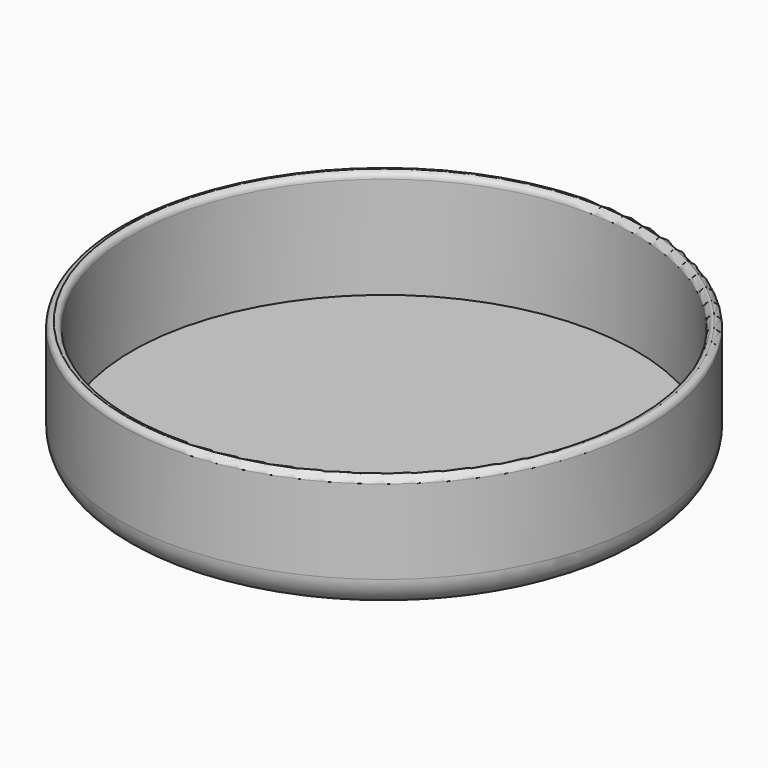
from build123d import *

# Parameters (mm, degrees)
F0_R     = 44
F1_DEPTH = 20
F2_T     = -2
F3_R     = 1
F4_R     = 0.99999
F5_R     = 5


# Not quite as in the source:
# - a fillet or chamfer is up to 0.001 mm smaller than in the source, because OpenCascade refuses the exact size


with BuildPart() as f1:
    # F0 (on Top) → F1 (new body)
    with BuildSketch(Plane.XY):
        Circle(F0_R)
    extrude(amount=F1_DEPTH)

    # F2
    f2_openings = [f1.faces().sort_by_distance(p)[0] for p in [
        (0, 0, 20),
    ]]
    offset(amount=F2_T, openings=f2_openings)

    # F3
    f3_edges = [f1.edges().sort_by_distance(p)[0] for p in [
        (-42, 0, 20),
    ]]
    fillet(f3_edges, radius=F3_R)

    # F4 (radius 1 in the source; OpenCascade refuses exactly that, so slightly less here)
    f4_edges = [f1.edges().sort_by_distance(p)[0] for p in [
        (-44, 0, 20),
    ]]
    fillet(f4_edges, radius=F4_R)

    # F5
    f5_edges = [f1.edges().sort_by_distance(p)[0] for p in [
        (-44, 0, 0),
    ]]
    fillet(f5_edges, radius=F5_R)


solid = f1.part
